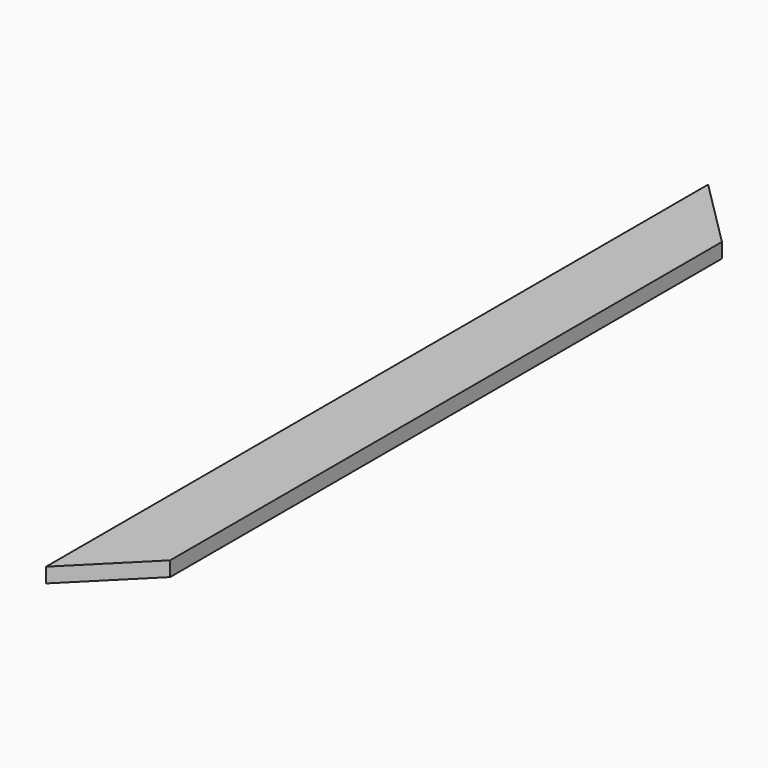
from build123d import *

# Parameters (mm, degrees)
F0_W     = 88.9
F0_H     = 1066.8
F1_DEPTH = 19.05
F2_SIZE  = 88.89999
F3_SIZE  = 88.89999


# Not quite as in the source:
# - a fillet or chamfer is up to 0.001 mm smaller than in the source, because OpenCascade refuses the exact size


with BuildPart() as f1:
    # F0 (on Top) → F1 (new body)
    with BuildSketch(Plane.XY):
        with Locations((-52.413374114, 471.9619610548)):
            Rectangle(F0_W, F0_H)
    extrude(amount=F1_DEPTH)

    # F2 (size 88.9 in the source; OpenCascade refuses exactly that, so slightly less here)
    f2_edges = [f1.edges().sort_by_distance(p)[0] for p in [
        (-7.963374, -61.438039, 9.525),
    ]]
    chamfer(f2_edges, length=F2_SIZE)

    # F3 (size 88.9 in the source; OpenCascade refuses exactly that, so slightly less here)
    f3_edges = [f1.edges().sort_by_distance(p)[0] for p in [
        (-7.963374, 1005.361961, 9.525),
    ]]
    chamfer(f3_edges, length=F3_SIZE)


solid = f1.part
